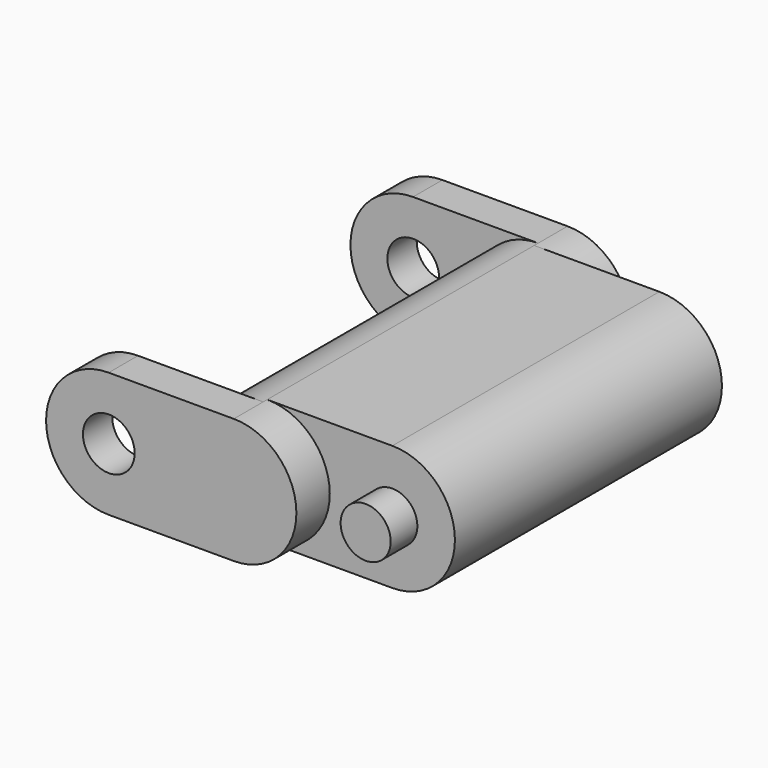
from build123d import *
from build123d import SkipClean  # not in build123d's __all__

# Parameters (mm, degrees)
F1_DEPTH  = 10
F2_DEPTH  = 12.5
F3_DEPTH  = 10.3
F4_R      = 1.5
F5_DEPTH  = 2
F4_R_2    = 1.55
F6_DEPTH  = 5
F7_R      = 1.5
F8_DEPTH  = 2
F7_R_2    = 1.55
F9_DEPTH  = 5
F11_DEPTH = 12.5


with BuildPart() as f1:
    # F0 (on Front) → F1 (new body, symmetric)
    with BuildSketch(Plane.XZ):
        with BuildLine():
            ThreePointArc((0, -3.75), (2.6516504294, -2.6516504294), (3.75, 0))
            ThreePointArc((3.75, 0), (2.6516504294, 2.6516504294), (0, 3.75))
            ThreePointArc((0, 3.75), (-2.6516504294, 2.6516504294), (-3.75, 0))
            ThreePointArc((-3.75, 0), (-2.6516504294, -2.6516504294), (0, -3.75))
        make_face()
        with BuildLine():
            ThreePointArc((0, 3.75), (2.6516504294, 2.6516504294), (3.75, 0))
            ThreePointArc((3.75, 0), (4.8483495706, 2.6516504294), (7.5, 3.75))
            Line((7.5, 3.75), (0, 3.75))
        make_face()
        with BuildLine():
            ThreePointArc((7.5, 3.75), (4.8483495706, 2.6516504294), (3.75, 0))
            ThreePointArc((3.75, 0), (4.8483495706, -2.6516504294), (7.5, -3.75))
            ThreePointArc((7.5, -3.75), (10.1516504294, -2.6516504294), (11.25, 0))
            ThreePointArc((11.25, 0), (10.1516504294, 2.6516504294), (7.5, 3.75))
        make_face()
        with BuildLine():
            ThreePointArc((7.5, -3.75), (4.8483495706, -2.6516504294), (3.75, 0))
            ThreePointArc((3.75, 0), (2.6516504294, -2.6516504294), (0, -3.75))
            Line((0, -3.75), (7.5, -3.75))
        make_face()
    extrude(amount=F1_DEPTH, both=True)

    # F0 (on Front) → F2 (join, symmetric)
    with BuildSketch(Plane.XZ):
        with BuildLine():
            ThreePointArc((-7.5, -3.75), (-4.8483495706, -2.6516504294), (-3.75, 0))
            ThreePointArc((-3.75, 0), (-4.8483495706, 2.6516504294), (-7.5, 3.75))
            ThreePointArc((-7.5, 3.75), (-11.25, 0), (-7.5, -3.75))
        make_face()
        with BuildLine():
            ThreePointArc((-3.75, 0), (-2.6516504294, 2.6516504294), (0, 3.75))
            Line((0, 3.75), (-7.5, 3.75))
            ThreePointArc((-7.5, 3.75), (-4.8483495706, 2.6516504294), (-3.75, 0))
        make_face()
        with BuildLine():
            ThreePointArc((0, -3.75), (2.6516504294, -2.6516504294), (3.75, 0))
            ThreePointArc((3.75, 0), (2.6516504294, 2.6516504294), (0, 3.75))
            ThreePointArc((0, 3.75), (-2.6516504294, 2.6516504294), (-3.75, 0))
            ThreePointArc((-3.75, 0), (-2.6516504294, -2.6516504294), (0, -3.75))
        make_face()
        with BuildLine():
            Line((-7.5, -3.75), (0, -3.75))
            ThreePointArc((0, -3.75), (-2.6516504294, -2.6516504294), (-3.75, 0))
            ThreePointArc((-3.75, 0), (-4.8483495706, -2.6516504294), (-7.5, -3.75))
        make_face()
    extrude(amount=F2_DEPTH, both=True)

    # F0 (on Front) → F3 (cut, symmetric)
    with BuildSketch(Plane.XZ):
        with BuildLine():
            ThreePointArc((-7.5, -3.75), (-4.8483495706, -2.6516504294), (-3.75, 0))
            ThreePointArc((-3.75, 0), (-4.8483495706, 2.6516504294), (-7.5, 3.75))
            ThreePointArc((-7.5, 3.75), (-11.25, 0), (-7.5, -3.75))
        make_face()
        with BuildLine():
            Line((-7.5, -3.75), (0, -3.75))
            ThreePointArc((0, -3.75), (-2.6516504294, -2.6516504294), (-3.75, 0))
            ThreePointArc((-3.75, 0), (-4.8483495706, -2.6516504294), (-7.5, -3.75))
        make_face()
        with BuildLine():
            ThreePointArc((-3.75, 0), (-2.6516504294, 2.6516504294), (0, 3.75))
            Line((0, 3.75), (-7.5, 3.75))
            ThreePointArc((-7.5, 3.75), (-4.8483495706, 2.6516504294), (-3.75, 0))
        make_face()
    with SkipClean():  # cleaning this boolean's faces spoils the solid; the shape is the same uncleaned
        extrude(amount=F3_DEPTH, both=True, mode=Mode.SUBTRACT)

    # F4 (on face) → F5 (join)
    with BuildSketch(Plane.XZ.offset(10)):
        with Locations((7.5, 0)):
            Circle(F4_R)
    extrude(amount=F5_DEPTH)

    # F4 (on face) → F6 (cut)
    with BuildSketch(Plane.XZ.offset(10)):
        with Locations((-7.4913557619, 0)):
            Circle(F4_R_2)
    extrude(amount=F6_DEPTH, mode=Mode.SUBTRACT)

    # F7 (on face) → F8 (join)
    with BuildSketch(Plane(origin=(0, 10, 0), x_dir=(-1, 0, 0), z_dir=(0, 1, 0))):
        with Locations((-7.5, 0)):
            Circle(F7_R)
    extrude(amount=F8_DEPTH)

    # F7 (on face) → F9 (cut)
    with BuildSketch(Plane(origin=(0, 10, 0), x_dir=(-1, 0, 0), z_dir=(0, 1, 0))):
        with Locations((7.4891448021, 0)):
            Circle(F7_R_2)
    extrude(amount=F9_DEPTH, mode=Mode.SUBTRACT)

    # F10 (on Top) → F11 (cut, symmetric)
    with BuildSketch(Plane.XY):
        Polygon((-3.2, -10.3), (-3.2, 0), (-3.2, 10.3), (-14.7820527132, 10.3), (-14.7820527132, -10.3), align=None)
    extrude(amount=F11_DEPTH, both=True, mode=Mode.SUBTRACT)


solid = f1.part
